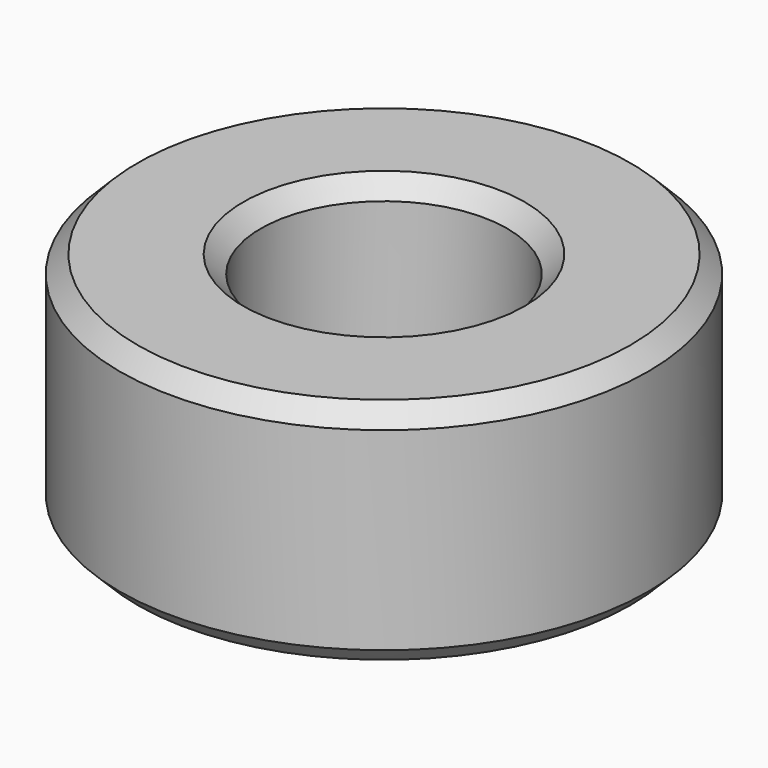
from build123d import *

# Parameters (mm, degrees)
F0_R     = 7.5
F0_R_2   = 3.5
F1_DEPTH = 6.5
F0_R_3   = 3
F2_DEPTH = 1.5
F3_SIZE  = 0.49999


# Not quite as in the source:
# - a fillet or chamfer is up to 0.001 mm smaller than in the source, because OpenCascade refuses the exact size


with BuildPart() as f1:
    # F0 (on Top) → F1 (new body)
    with BuildSketch(Plane.XY):
        with Locations((-72.2782313824, 42.1795584261)):
            Circle(F0_R)
        with Locations((-72.2782313824, 42.1795584261)):
            Circle(F0_R_2, mode=Mode.SUBTRACT)
    extrude(amount=F1_DEPTH)

    # F0 (on Top) → F2 (join)
    with BuildSketch(Plane.XY):
        with Locations((-72.2782313824, 42.1795584261)):
            Circle(F0_R_2)
        with Locations((-72.2782313824, 42.1795584261)):
            Circle(F0_R_3, mode=Mode.SUBTRACT)
    extrude(amount=F2_DEPTH)

    # F3 (size 0.5 in the source; OpenCascade refuses exactly that, so slightly less here)
    f3_edges = [f1.edges().sort_by_distance(p)[0] for p in [
        (-79.778231, 42.179558, 6.5),
        (-75.778231, 42.179558, 6.5),
        (-75.278231, 42.179558, 1.5),
        (-79.778231, 42.179558, 0),
    ]]
    chamfer(f3_edges, length=F3_SIZE)


solid = f1.part
